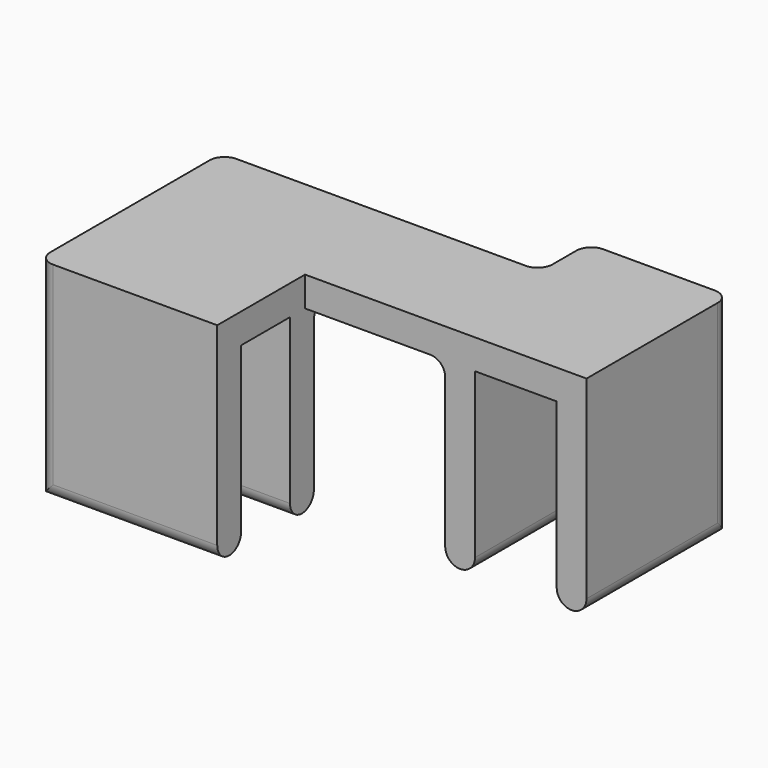
from build123d import *

# Parameters (mm, degrees)
F2_DEPTH = 10
F3_W     = 60
F3_H     = 10
F3_W_2   = 10
F3_H_2   = 60
F4_DEPTH = 60
F5_R     = 4.99999


# Not quite as in the source:
# - a fillet or chamfer is up to 0.001 mm smaller than in the source, because OpenCascade refuses the exact size


with BuildPart() as f2:
    # F1 (on Top) → F2 (new body)
    with BuildSketch(Plane.XY):
        Polygon((-11, 65.8), (-11, -11), (49, -11), (49, 25.8), (143.4, 25.8), (143.4, 85.8), (96, 85.8), (96, 65.8), align=None)
    extrude(amount=F2_DEPTH)

    # F3 (on face) → F4 (join)
    with BuildSketch(Plane(origin=(0, 0, 0), x_dir=(1, 0, 0), z_dir=(0, 0, -1))):
        with Locations((19, 6)):
            Rectangle(F3_W, F3_H)
        with Locations((19, -24.5)):
            Rectangle(F3_W, F3_H)
        with Locations((101, -55.8)):
            Rectangle(F3_W_2, F3_H_2)
        with Locations((138.4, -55.8)):
            Rectangle(F3_W_2, F3_H_2)
    extrude(amount=F4_DEPTH)

    # F5 (radius 5 in the source; OpenCascade refuses exactly that, so slightly less here)
    f5_edges = [f2.edges().sort_by_distance(p)[0] for p in [
        (96, 65.8, 5),
        (96, 85.8, -25),
        (143.4, 85.8, -25),
        (-11, 65.8, 5),
        (-11, 29.5, -30),
        (-11, -11, -25),
        (119.7, 85.8, 0),
        (42.5, 65.8, 0),
        (-11, 47.65, 0),
        (-11, 9.25, 0),
        (133.4, 55.8, -60),
        (106, 55.8, -60),
        (96, 55.8, -60),
        (143.4, 55.8, -60),
        (19, 29.5, 0),
        (19, 29.5, -60),
        (19, -11, -60),
        (19, -1, -60),
        (19, 19.5, -60),
        (96, 45.8, 0),
    ]]
    fillet(f5_edges, radius=F5_R)


solid = f2.part
